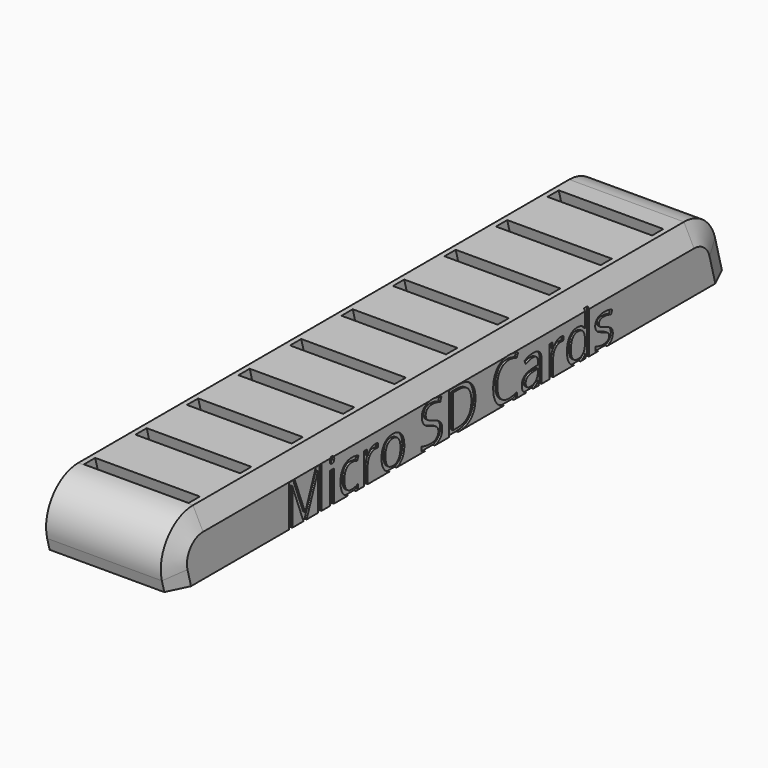
from build123d import *

# Parameters (mm, degrees)
F2_DEPTH      = 5.2
F4_DEPTH      = 1.5
F6_R          = 4
F7_SIZE2      = 2
F7_SIZE       = 1
F8_TEXT_SIZE  = 5.7633737937
F9_DEPTH      = 0.2
F10_TEXT_SIZE = 5.7633737937
F11_DEPTH     = 0.2


# Not quite as in the source:
# - Text() gives the source's letters only with a copy of the font that has no kerning and outlines rounded to 1/6400 em; it was checked with that copy


with BuildPart() as f2:
    # F1 (on Right) → F2 (new body)
    with BuildSketch(Plane.YZ):
        Polygon((-9.2644166164, 6.1496291314), (-7.6166284568, 0), (61.6536673639, 0), (60.0058792044, 6.1496291314), (55.0058792044, 6.1496291314), (56.2063514519, 1.6694057109), (54.9023515864, 1.32), (53.6082563609, 6.1496291314), (48.6082563609, 6.1496291314), (49.8087286083, 1.6694057109), (48.5047287428, 1.32), (47.2106335173, 6.1496291314), (42.2106335173, 6.1496291314), (43.4111057647, 1.6694057109), (42.1071058993, 1.32), (40.8130106737, 6.1496291314), (35.8130106737, 6.1496291314), (37.0134829212, 1.6694057109), (35.7094830557, 1.32), (34.4153878302, 6.1496291314), (29.4153878302, 6.1496291314), (30.6158600776, 1.6694057109), (29.3118602122, 1.32), (28.0177649866, 6.1496291314), (23.0177649866, 6.1496291314), (24.2182372341, 1.6694057109), (22.9142373686, 1.32), (21.6201421431, 6.1496291314), (16.6201421431, 6.1496291314), (17.8206143905, 1.6694057109), (16.516614525, 1.32), (15.2225192995, 6.1496291314), (10.2225192995, 6.1496291314), (11.422991547, 1.6694057109), (10.1189916815, 1.32), (8.824896456, 6.1496291314), (3.824896456, 6.1496291314), (5.0253687034, 1.6694057109), (3.7213688379, 1.32), (2.4272736124, 6.1496291314), (-2.5727263876, 6.1496291314), (-1.3722541401, 1.6694057109), (-2.6762540056, 1.32), (-3.9703492311, 6.1496291314), align=None)
    extrude(amount=F2_DEPTH)

    # F3 (on face) → F4 (join)
    with BuildSketch(Plane.YZ.offset(5.2)):
        Polygon((-3.9703492311, 6.1496291314), (-9.2644166164, 6.1496291314), (-7.6166284568, 0), (61.6536673639, 0), (60.0058792044, 6.1496291314), (55.0058792044, 6.1496291314), (56.2063514519, 1.6694057109), (54.9023515864, 1.32), (53.6082563609, 6.1496291314), (48.6082563609, 6.1496291314), (49.8087286083, 1.6694057109), (48.5047287428, 1.32), (47.2106335173, 6.1496291314), (42.2106335173, 6.1496291314), (43.4111057647, 1.6694057109), (42.1071058993, 1.32), (40.8130106737, 6.1496291314), (35.8130106737, 6.1496291314), (37.0134829212, 1.6694057109), (35.7094830557, 1.32), (34.4153878302, 6.1496291314), (29.4153878302, 6.1496291314), (30.6158600776, 1.6694057109), (29.3118602122, 1.32), (28.0177649866, 6.1496291314), (23.0177649866, 6.1496291314), (24.2182372341, 1.6694057109), (22.9142373686, 1.32), (21.6201421431, 6.1496291314), (16.6201421431, 6.1496291314), (17.8206143905, 1.6694057109), (16.516614525, 1.32), (15.2225192995, 6.1496291314), (10.2225192995, 6.1496291314), (11.422991547, 1.6694057109), (10.1189916815, 1.32), (8.824896456, 6.1496291314), (3.824896456, 6.1496291314), (5.0253687034, 1.6694057109), (3.7213688379, 1.32), (2.4272736124, 6.1496291314), (-2.5727263876, 6.1496291314), (-1.3722541401, 1.6694057109), (-2.6762540056, 1.32), align=None)
        Polygon((-2.5727263876, 6.1496291314), (-3.9703492311, 6.1496291314), (-2.6762540056, 1.32), (-1.3722541401, 1.6694057109), align=None)
        Polygon((3.824896456, 6.1496291314), (2.4272736124, 6.1496291314), (3.7213688379, 1.32), (5.0253687034, 1.6694057109), align=None)
        Polygon((10.2225192995, 6.1496291314), (8.824896456, 6.1496291314), (10.1189916815, 1.32), (11.422991547, 1.6694057109), align=None)
        Polygon((16.6201421431, 6.1496291314), (15.2225192995, 6.1496291314), (16.516614525, 1.32), (17.8206143905, 1.6694057109), align=None)
        Polygon((23.0177649866, 6.1496291314), (21.6201421431, 6.1496291314), (22.9142373686, 1.32), (24.2182372341, 1.6694057109), align=None)
        Polygon((29.4153878302, 6.1496291314), (28.0177649866, 6.1496291314), (29.3118602122, 1.32), (30.6158600776, 1.6694057109), align=None)
        Polygon((37.0134829212, 1.6694057109), (35.8130106737, 6.1496291314), (34.4153878302, 6.1496291314), (35.7094830557, 1.32), align=None)
        Polygon((43.4111057647, 1.6694057109), (42.2106335173, 6.1496291314), (40.8130106737, 6.1496291314), (42.1071058993, 1.32), align=None)
        Polygon((49.8087286083, 1.6694057109), (48.6082563609, 6.1496291314), (47.2106335173, 6.1496291314), (48.5047287428, 1.32), align=None)
        Polygon((56.2063514519, 1.6694057109), (55.0058792044, 6.1496291314), (53.6082563609, 6.1496291314), (54.9023515864, 1.32), align=None)
    extrude(amount=F4_DEPTH)

    # F5: F2 across face


with BuildPart() as f2_1:
    add(f2.part)
    add(f2.part.mirror(Plane(origin=(0, 26.205741201, 2.9402994114), x_dir=(0, 1, 0), z_dir=(-1, 0, 0))))

    # F6
    f6_edges = [f2_1.edges().sort_by_distance(p)[0] for p in [
        (0, 60.005879, 6.149629),
        (0, -9.264417, 6.149629),
    ]]
    fillet(f6_edges, radius=F6_R)

    # F7
    f7_edges = [f2_1.edges().sort_by_distance(p)[0] for p in [
        (-6.7, 26.442528, 6.149629),
        (6.7, 26.442528, 6.149629),
    ]]
    f7_side = f2_1.faces().sort_by_distance((0, 26.642587, 6.149629))[0]
    chamfer(f7_edges, length=F7_SIZE, length2=F7_SIZE2, reference=f7_side)

    # F8 (on face) → F9 (cut)
    with BuildSketch(Plane.YZ.offset(6.7)):
        with Locations((6.0370329891, 0)):
            Text('Micro SD Cards', F8_TEXT_SIZE, font='Open Sans', text_align=(TextAlign.LEFT, TextAlign.BOTTOM))
    extrude(amount=-F9_DEPTH, mode=Mode.SUBTRACT)

    # F10 (on face) → F11 (cut)
    with BuildSketch(Plane(origin=(-6.7, 0, 0), x_dir=(0, -1, 0), z_dir=(-1, 0, 0))):
        with Locations((-46.8480231384, 0)):
            Text('Micro SD Cards', F10_TEXT_SIZE, font='Open Sans', text_align=(TextAlign.LEFT, TextAlign.BOTTOM))
    extrude(amount=-F11_DEPTH, mode=Mode.SUBTRACT)


solid = f2_1.part
